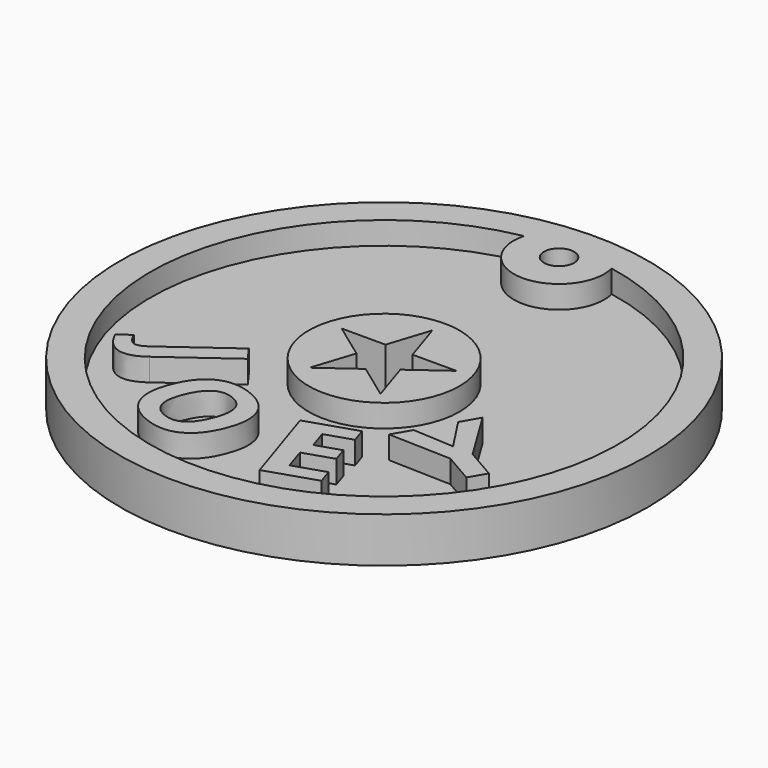
from build123d import *

# Parameters (mm, degrees)
F0_R           = 17.5
F1_DEPTH       = 3
F2_R           = 5
F3_DEPTH       = 1.5
F4_R           = 1
F5_DEPTH       = 3.001
F7_DEPTH       = 3.001
F8_TEXT_SIZE   = 7.6388888889
F8_TEXT_SIZE_2 = 8.3333333333
F9_DEPTH       = 1.5


# Not quite as in the source:
# - Text() gives the source's letters only with a copy of the font that has no kerning and outlines rounded to 1/6400 em; it was checked with that copy


with BuildPart() as f1:
    # F0 (on Top) → F1 (new body)
    with BuildSketch(Plane.XY):
        Circle(F0_R)
    extrude(amount=F1_DEPTH)

    # F2 (on face) → F3 (cut)
    with BuildSketch(Plane.XY.offset(3)):
        with BuildLine():
            ThreePointArc((2.9112925406, 15.224137931), (0, 11.5), (-2.9112925406, 15.224137931))
            ThreePointArc((-2.9112925406, 15.224137931), (0, -15.5), (2.9112925406, 15.224137931))
        make_face()
        Circle(F2_R, mode=Mode.SUBTRACT)
    extrude(amount=-F3_DEPTH, mode=Mode.SUBTRACT)

    # F4 (on face) → F5 (cut, through all)
    with BuildSketch(Plane.XY.offset(3)):
        with Locations((0, 14.5)):
            Circle(F4_R)
    extrude(amount=-F5_DEPTH, mode=Mode.SUBTRACT)

    # F6 (on face) → F7 (cut, through all)
    with BuildSketch(Plane.XY.offset(3)):
        Polygon((0.8980559532, 1.2360679775), (0, 4), (-0.8980559532, 1.2360679775), (-3.8042260652, 1.2360679775), (-1.453085056, -0.472135955), (-2.3511410092, -3.2360679775), (0, -1.527864045), (2.3511410092, -3.2360679775), (1.453085056, -0.472135955), (3.8042260652, 1.2360679775), align=None)
    extrude(amount=-F7_DEPTH, mode=Mode.SUBTRACT)

    # F8 (on face) → F9 (join)
    with BuildSketch(Plane.XY.offset(1.5)):
        with Locations(Location((-10.9665189805, -6.1721517535), (0, 0, -54))):
            Text('J', F8_TEXT_SIZE, font='Open Sans', font_style=FontStyle.BOLD, text_align=(TextAlign.LEFT, TextAlign.BOTTOM))
        with Locations(Location((-8.3453669569, -11.7277392827), (0, 0, -22))):
            Text('O', F8_TEXT_SIZE_2, font='Open Sans', font_style=FontStyle.BOLD, text_align=(TextAlign.LEFT, TextAlign.BOTTOM))
        Polygon((4.215952402, -7.0952463862), (2.4878282242, -7.6567479691), (2.8073067315, -8.6400017112), (4.5354309092, -8.0785001283), align=None)
        Polygon((2.8073067315, -8.6400017112), (2.4878282242, -7.6567479691), (0.9578408208, -8.1538710115), (2.7962505178, -13.8119142705), (6.054362099, -12.7532896453), (5.7324693965, -11.7626057741), (3.6743236542, -12.4313378635), (3.2003366498, -10.9725558632), (5.1160715856, -10.3500958498), (4.7965930784, -9.3668421077), (3.2108797072, -9.8820716146), (2.8808581426, -9.9893021211), (2.4772851669, -8.7472322177), align=None)
        Polygon((3.2108797072, -9.8820716146), (2.8073067315, -8.6400017112), (2.4772851669, -8.7472322177), (2.8808581426, -9.9893021211), align=None)
        with Locations(Location((10.6891342988, -9.4858763055), (0, 0, 60))):
            Text('Y', F8_TEXT_SIZE_2, font='Open Sans', font_style=FontStyle.BOLD, text_align=(TextAlign.LEFT, TextAlign.BOTTOM))
    extrude(amount=F9_DEPTH)


solid = f1.part
